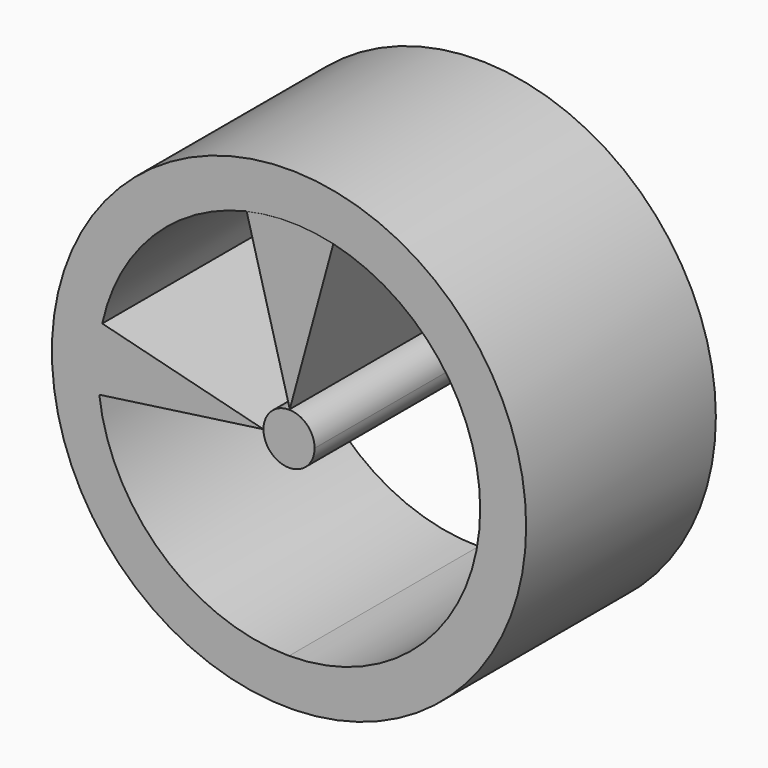
from build123d import *

# Parameters (mm, degrees)
F0_R     = 12.7
F1_DEPTH = 12.7
F2_DEPTH = 12.7
F4_DEPTH = 12.6492


# Not quite as in the source:
# - a feature of the source that left no trace in its solid (it failed there, or was rolled back) is left out


with BuildPart() as f1:
    # F0 (on Front) → F1 (new body)
    with BuildSketch(Plane.XZ):
        Circle(F0_R)
        with BuildLine():
            ThreePointArc((2.342264303, 9.9660302686), (8.0245582458, 6.3572341736), (10.2375759523, 0))
            ThreePointArc((10.2375759523, 0), (7.2390593788, -7.2390593788), (0, -10.2375759523))
            ThreePointArc((0, -10.2375759523), (-6.7907141872, -7.6612115365), (-10.1635578802, -1.2288419733))
            ThreePointArc((-10.1635578802, -1.2288419733), (-10.2262516737, 0.4813918215), (-10.003175629, 2.178173252))
            ThreePointArc((-10.003175629, 2.178173252), (-7.2893862495, 7.1883801711), (-2.3175314223, 9.9718107426))
            ThreePointArc((-2.3175314223, 9.9718107426), (0.0126996975, 10.2375680753), (2.342264303, 9.9660302686))
        make_face(mode=Mode.SUBTRACT)
    extrude(amount=F1_DEPTH)

    # F0 (on Front) → F2 (join)
    with BuildSketch(Plane.XZ):
        with BuildLine():
            ThreePointArc((-10.003175629, 2.178173252), (-10.2262516737, 0.4813918215), (-10.1635578802, -1.2288419733))
            Line((-10.1635578802, -1.2288419733), (-1.3697025857, 0))
            Line((-1.3697025857, 0), (-10.003175629, 2.178173252))
        make_face()
    extrude(amount=F2_DEPTH)

    # F0 (on Front) → F4 (join)
    with BuildSketch(Plane.XZ):
        with BuildLine():
            Line((0, 1.3697025857), (2.342264303, 9.9660302686))
            ThreePointArc((2.342264303, 9.9660302686), (0.0126996975, 10.2375680753), (-2.3175314223, 9.9718107426))
            Line((-2.3175314223, 9.9718107426), (0, 1.3697025857))
        make_face()
    extrude(amount=F4_DEPTH)


with BuildPart() as f1b:
    # F0 (on Front) → F1, piece 2 (new body)
    with BuildSketch(Plane.XZ):
        with BuildLine():
            ThreePointArc((0, -1.3697025857), (0.9685259866, -0.9685259866), (1.3697025857, 0))
            ThreePointArc((1.3697025857, 0), (0.9685259866, 0.9685259866), (0, 1.3697025857))
            ThreePointArc((0, 1.3697025857), (-0.9685259866, 0.9685259866), (-1.3697025857, 0))
            ThreePointArc((-1.3697025857, 0), (-0.9685259866, -0.9685259866), (0, -1.3697025857))
        make_face()
    extrude(amount=F1_DEPTH)


solid = Compound([f1.part, f1b.part])
